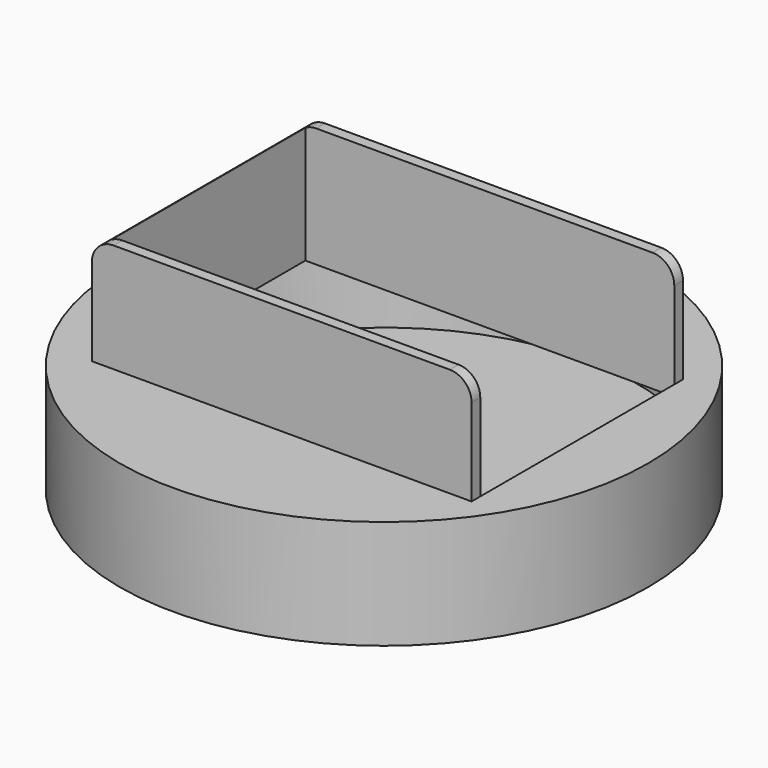
from build123d import *

# Parameters (mm, degrees)
F0_R        = 61.5660175878
F1_DEPTH    = 25.4
F2_W        = 88.528262917
F2_H        = 61.6074204445
F3_DEPTH    = 25.4
F4_T        = 2.54
F4_T3_DEPTH = 93.608262917
F4_T5_DEPTH = 66.6874204445
F5_T1_DEPTH = 87.0074204445
F6_R        = 5.08


# Not quite as in the source:
# - a fillet or chamfer that OpenCascade refuses, or shapes differently, is made with other operations: its cross-section is extruded or revolved along the edge and cut away or added
# - a shell that OpenCascade refuses in one call is made with other operations: the cavity is built on its own and cut out


with BuildPart() as f1:
    # F0 (on Top) → F1 (new body)
    with BuildSketch(Plane.XY):
        with Locations((-52.3894988, 0)):
            Circle(F0_R)
    extrude(amount=F1_DEPTH)

    # F2 (on face) → F3 (join)
    with BuildSketch(Plane.XY.offset(25.4)):
        with Locations((-50.8173767012, -0.9788312018)):
            Rectangle(F2_W, F2_H)
    extrude(amount=F3_DEPTH)

    # F4: shell of thickness 2.54, made by hand


with BuildPart() as f4_core1:
    # F4_t2: copy of F1
    add(f1.part)

    # the walls: a layer under each face that stays
    f4_faces = [f4_core1.faces().sort_by_distance(p)[0] for p in [
        (-113.9555163879, 0, 12.7),
        (-52.3894988, 0, 0),
        (-93.4335105253, -41.0440117252, 25.4),
        (-50.8173767012, 29.8248790205, 38.1),
        (-95.0815081596, -0.9788312018, 38.1),
        (-50.8173767012, -31.782541424, 38.1),
    ]]
    thicken(f4_faces, amount=-F4_T, mode=Mode.SUBTRACT)

    # F4_s4 → F4_t3 (cut)
    with BuildSketch(Plane.YZ.offset(-97.6215081596)):
        Polygon((29.8502790205, 25.4254), (29.8248790205, 22.86), (27.2848790205, 22.86), (27.2848790205, 25.4), align=None)
        Polygon((-31.807941424, 25.4254), (-31.782541424, 22.86), (-29.242541424, 22.86), (-29.242541424, 25.4), align=None)
    extrude(amount=F4_T3_DEPTH, mode=Mode.SUBTRACT)

    # F4_s6 → F4_t5 (cut)
    with BuildSketch(Plane.XZ.offset(-32.3648790205)):
        Polygon((-95.1069081596, 25.4254), (-95.0815081596, 22.86), (-92.5415081596, 22.86), (-92.5415081596, 25.4), align=None)
    extrude(amount=F4_T5_DEPTH, mode=Mode.SUBTRACT)


with BuildPart() as f1_1:
    add(f1.part)

    # what is left inside the walls is the cavity
    f4_cavity = [f4_core1.part.solids().sort_by_distance(p)[0] for p in [
        (-52.389499, -19.675339, 2.5654),
    ]]
    add(f4_cavity, mode=Mode.SUBTRACT)

    # F5: fillet of radius 5.08 on 1 edges, made by hand

    # F5_s2 → F5_t1 (cut)
    with BuildSketch(Plane.XZ.offset(-42.5248790205)):
        with BuildLine():
            ThreePointArc((-95.0815081596, 45.72), (-93.5936106081, 49.3121024484), (-90.0015081596, 50.8))
            Line((-90.0015081596, 50.8), (-95.0815081596, 50.8))
            Line((-95.0815081596, 50.8), (-95.0815081596, 45.72))
        make_face()
    extrude(amount=F5_T1_DEPTH, mode=Mode.SUBTRACT)

    # F6
    f6_edges = [f1_1.edges().sort_by_distance(p)[0] for p in [
        (-6.553245, -30.512541, 50.8),
        (-6.553245, 28.554879, 50.8),
    ]]
    fillet(f6_edges, radius=F6_R)


solid = f1_1.part
